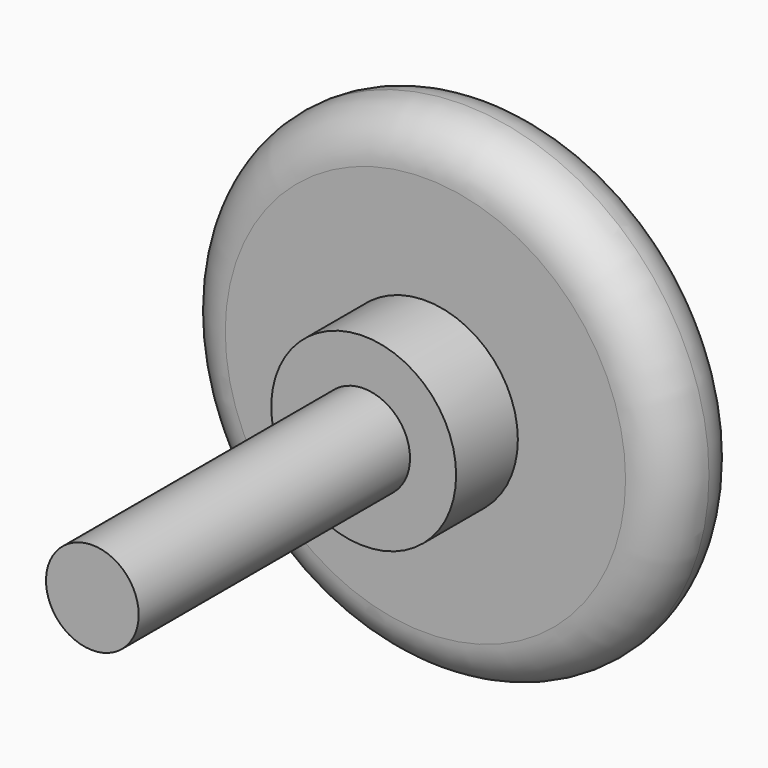
from build123d import *

# Parameters (mm, degrees)
F0_R     = 12.7
F1_DEPTH = 4.7752
F2_R     = 2.38759
F3_R     = 4.7625
F4_DEPTH = 3.9751
F5_R     = 2.3876
F6_DEPTH = 17.4752


# Not quite as in the source:
# - a fillet or chamfer is up to 0.001 mm smaller than in the source, because OpenCascade refuses the exact size


with BuildPart() as f1:
    # F0 (on Front) → F1 (new body)
    with BuildSketch(Plane.XZ):
        Circle(F0_R)
    extrude(amount=F1_DEPTH)

    # F2 (radius 2.3876 in the source; OpenCascade refuses exactly that, so slightly less here)
    f2_edges = [f1.edges().sort_by_distance(p)[0] for p in [
        (-12.7, 0, 0),
        (-12.7, -4.7752, 0),
    ]]
    fillet(f2_edges, radius=F2_R)

    # F3 (on face) → F4 (join, symmetric)
    with BuildSketch(Plane.XZ.offset(4.7752)):
        Circle(F3_R)
    extrude(amount=F4_DEPTH, both=True)

    # F5 (on face) → F6 (join)
    with BuildSketch(Plane.XZ.offset(8.7503)):
        Circle(F5_R)
    extrude(amount=F6_DEPTH)


solid = f1.part
